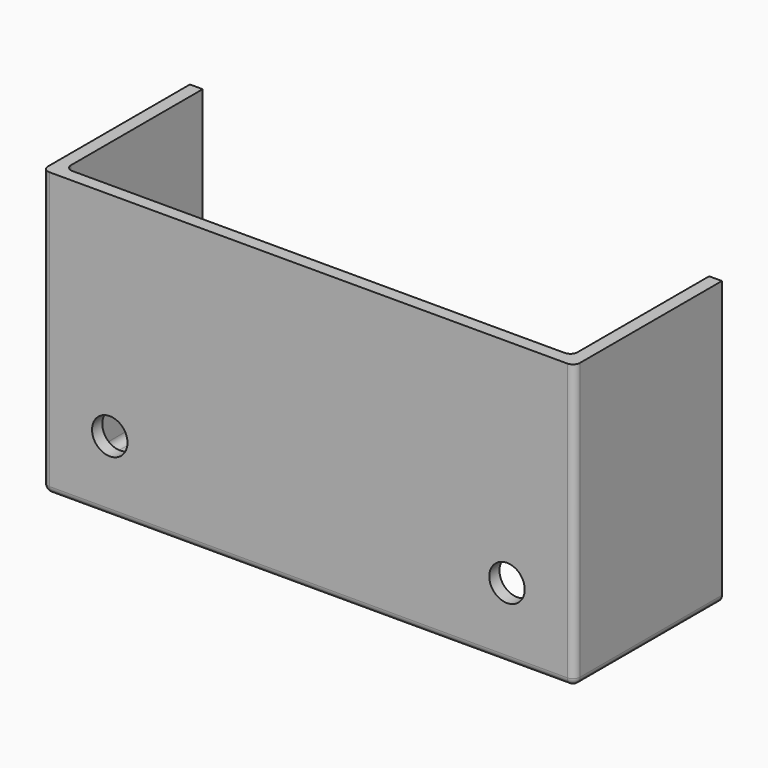
from build123d import *

# Parameters (mm, degrees)
F0_W      = 75
F0_H      = 26
F1_DEPTH  = 2
F2_W      = 75
F2_H      = 26
F2_W_2    = 71.4
F2_H_2    = 22.4
F3_DEPTH  = 38
F5_DEPTH  = 2
F6_R      = 2.5
F7_DEPTH  = 1.8
F8_W      = 36
F8_H      = 6
F9_DEPTH  = 1.8
F10_SIZE  = 1.79999
F11_W     = 71.4
F11_H     = 1.8
F12_DEPTH = 20
F13_R     = 3.125
F14_DEPTH = 10
F15_R     = 0.75
F16_R     = 1.65
F17_DEPTH = 40.001
F18_F1_R  = 1
F18_F2_R  = 1
F19_R     = 2.5
F20_DEPTH = 27.801


# Not quite as in the source:
# - a fillet or chamfer is up to 0.001 mm smaller than in the source, because OpenCascade refuses the exact size


with BuildPart() as f1:
    # F0 (on Top) → F1 (new body)
    with BuildSketch(Plane.XY):
        Rectangle(F0_W, F0_H)
    extrude(amount=F1_DEPTH)

    # F2 (on face) → F3 (join)
    with BuildSketch(Plane.XY.offset(2)):
        Rectangle(F2_W, F2_H)
        Rectangle(F2_W_2, F2_H_2, mode=Mode.SUBTRACT)
    extrude(amount=F3_DEPTH)

    # F4 (on face) → F5 (cut, through all)
    with BuildSketch(Plane(origin=(0, 0, 0), x_dir=(1, 0, 0), z_dir=(0, 0, -1))):
        with BuildLine():
            Line((-22.35, 2.6110342778), (-22.35, -2.6110342778))
            ThreePointArc((-22.35, -2.6110342778), (-15, -7.8), (-7.65, -2.6110342778))
            Line((-7.65, -2.6110342778), (-7.65, 2.6110342778))
            ThreePointArc((-7.65, 2.6110342778), (-15, 7.8), (-22.35, 2.6110342778))
        make_face()
        with BuildLine():
            ThreePointArc((22.35, 2.6110342778), (15, 7.8), (7.65, 2.6110342778))
            Line((7.65, 2.6110342778), (7.65, -2.6110342778))
            ThreePointArc((7.65, -2.6110342778), (15, -7.8), (22.35, -2.6110342778))
            Line((22.35, -2.6110342778), (22.35, 2.6110342778))
        make_face()
    extrude(amount=-F5_DEPTH, mode=Mode.SUBTRACT)

    # F6 (on face) → F7 (cut, through all)
    with BuildSketch(Plane(origin=(0, 13, 0), x_dir=(-1, 0, 0), z_dir=(0, 1, 0))):
        with Locations((28, 10)):
            Circle(F6_R)
        with Locations((-28, 10)):
            Circle(F6_R)
    extrude(amount=-F7_DEPTH, mode=Mode.SUBTRACT)

    # F8 (on face) → F9 (join)
    with BuildSketch(Plane(origin=(0, 13, 0), x_dir=(-1, 0, 0), z_dir=(0, 1, 0))):
        with Locations((0, 10)):
            Rectangle(F8_W, F8_H)
    extrude(amount=F9_DEPTH)

    # F10 (size 1.8 in the source; OpenCascade refuses exactly that, so slightly less here)
    f10_edges = [f1.edges().sort_by_distance(p)[0] for p in [
        (0, 14.8, 7),
    ]]
    chamfer(f10_edges, length=F10_SIZE)

    # F11 (on face) → F12 (cut)
    with BuildSketch(Plane.XY.offset(40)):
        with Locations((0, 12.1)):
            Rectangle(F11_W, F11_H)
    extrude(amount=-F12_DEPTH, mode=Mode.SUBTRACT)

    # F13 (on face) → F14 (join)
    with BuildSketch(Plane.XY.offset(2)):
        Circle(F13_R)
    extrude(amount=F14_DEPTH)

    # F15
    f15_edges = [f1.edges().sort_by_distance(p)[0] for p in [
        (-3.125, 0, 12),
    ]]
    fillet(f15_edges, radius=F15_R)

    # F16 (on face) → F17 (cut, through all)
    with BuildSketch(Plane(origin=(0, 0, 0), x_dir=(1, 0, 0), z_dir=(0, 0, -1))):
        Circle(F16_R)
    extrude(amount=-F17_DEPTH, mode=Mode.SUBTRACT)

    # F18: fillet of radius 1 on 14 edges, made by hand

    # F18_f1
    f18_f1_edges = [f1.edges().sort_by_distance(p)[0] for p in [
        (-37.5, -13, 20),
        (37.5, -13, 20),
        (0, -13, 0),
        (37.5, 0, 0),
        (-37.5, 0, 0),
        (0, 11.2, 20),
    ]]
    fillet(f18_f1_edges, radius=F18_F1_R)

    # F18_f2
    f18_f2_edges = [f1.edges().sort_by_distance(p)[0] for p in [
        (-35.7, -11.2, 21),
        (35.7, -11.2, 21),
        (0, -11.2, 2),
        (35.7, 0, 2),
        (-35.7, 0, 2),
        (0, 11.2, 2),
        (35.7, 11.2, 10.5),
        (-35.7, 11.2, 10.5),
        (-35.7, 11.4928932188, 19.7071067812),
        (35.7, 11.4928932188, 19.7071067812),
    ]]
    fillet(f18_f2_edges, radius=F18_F2_R)

    # F19 (on face) → F20 (cut, through all)
    with BuildSketch(Plane.XZ.offset(13)):
        with Locations((28, 10)):
            Circle(F19_R)
        with Locations((-28, 10)):
            Circle(F19_R)
    extrude(amount=-F20_DEPTH, mode=Mode.SUBTRACT)


solid = f1.part
